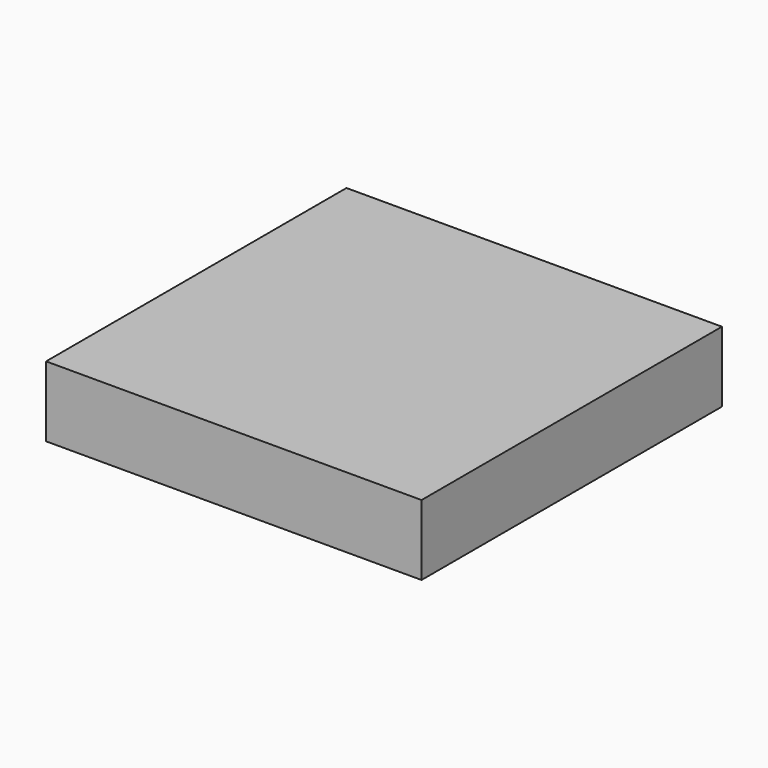
from build123d import *

# Parameters (mm, degrees)
F0_W     = 76.2
F0_H     = 76.2
F0_W_2   = 50.8
F0_H_2   = 50.8
F1_DEPTH = 7.14375


# Not quite as in the source:
# - a length typed as a fraction of an inch, garbled in the dataset ("3 / 203.2 mm" for 3/8 in), is restored


with BuildPart() as f1:
    # F0 (on Top) → F1 (new body, symmetric)
    with BuildSketch(Plane.XY):
        Rectangle(F0_W, F0_H)
        Rectangle(F0_W_2, F0_H_2, mode=Mode.SUBTRACT)
        Rectangle(F0_W_2, F0_H_2)
    extrude(amount=F1_DEPTH, both=True)


solid = f1.part
